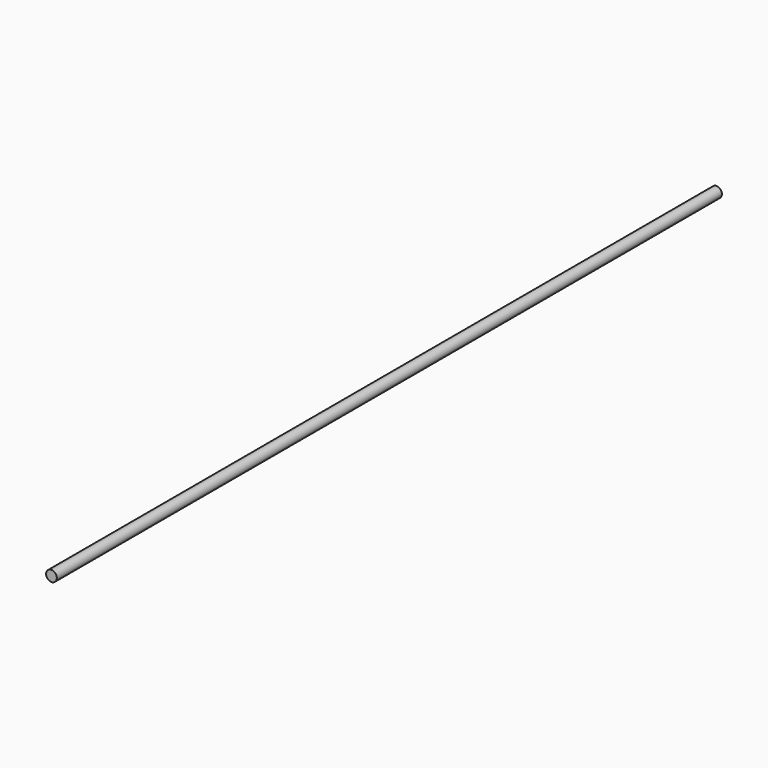
from build123d import *

# Parameters (mm, degrees)
F1_R     = 1.27
F2_DEPTH = 196.85


# Not quite as in the source:
# - a variable given as a bare number and used for a length is read in inches; the dataset says mm whatever the document's units were


with BuildPart() as f2:
    # F1 (on Front) → F2 (new body)
    with BuildSketch(Plane.XZ):
        Circle(F1_R)
    extrude(amount=F2_DEPTH)


solid = f2.part
